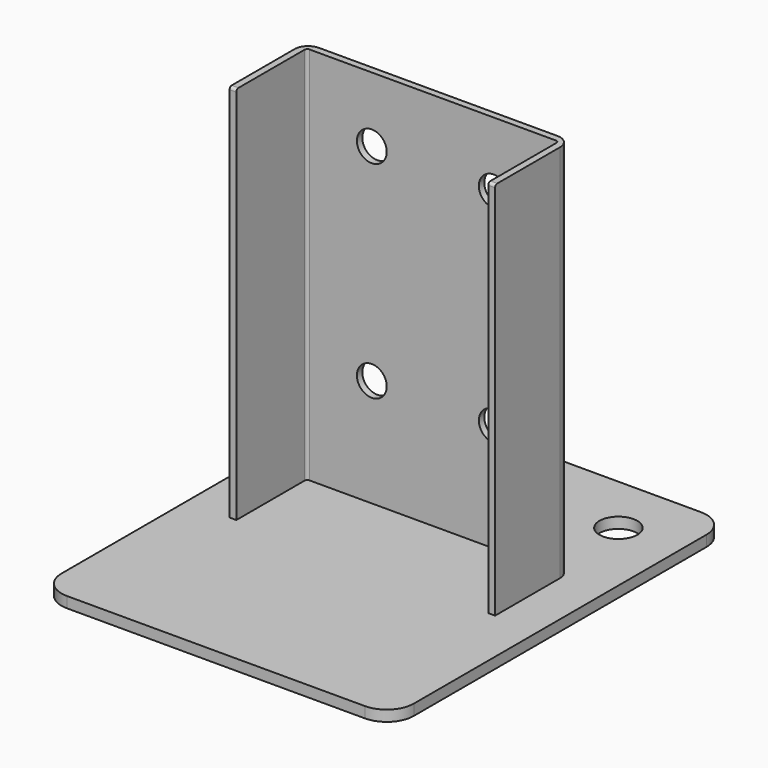
from build123d import *

# Parameters (mm, degrees)
F0_W     = 130
F0_H     = 155
F1_DEPTH = 4
F2_R     = 10
F4_DEPTH = 140
F5_R     = 5
F6_R     = 1
F7_R     = 1
F9_D     = 14
F11_D    = 11


# Not quite as in the source:
# - a feature names something its author has since deleted; it is built from what else it names


with BuildPart() as f1:
    # F0 (on Top) → F1 (new body)
    with BuildSketch(Plane.XY):
        with Locations((-65, 36.8233056366)):
            Rectangle(F0_W, F0_H)
    extrude(amount=F1_DEPTH)

    # F2
    f2_edges = [f1.edges().sort_by_distance(p)[0] for p in [
        (0, -40.676694, 2),
        (0, 114.323306, 2),
        (-130, 114.323306, 2),
        (-130, -40.676694, 2),
    ]]
    fillet(f2_edges, radius=F2_R)

    # F3 (on face) → F4 (join)
    with BuildSketch(Plane.XY.offset(4)):
        Polygon((-16, 26.8233056366), (-16, 61.8233056366), (-114, 61.8233056366), (-114, 26.8233056366), (-111.5, 26.8233056366), (-111.5, 59.3233056366), (-18.5, 59.3233056366), (-18.5, 26.8233056366), align=None)
    extrude(amount=F4_DEPTH)

    # F5
    f5_edges = [f1.edges().sort_by_distance(p)[0] for p in [
        (-114, 61.823306, 74),
        (-16, 61.823306, 74),
    ]]
    fillet(f5_edges, radius=F5_R)

    # F6
    f6_edges = [f1.edges().sort_by_distance(p)[0] for p in [
        (-18.5, 59.323306, 74),
        (-111.5, 59.323306, 74),
    ]]
    fillet(f6_edges, radius=F6_R)

    # F7
    f7_edges = [f1.edges().sort_by_distance(p)[0] for p in [
        (-112.75, 26.823306, 144),
        (-17.25, 26.823306, 144),
    ]]
    fillet(f7_edges, radius=F7_R)

    # F9 (through all)
    with Locations(Plane.XY.offset(4)):
        with Locations((-22.5, 91.8233056366), (-65, 91.8233056366), (-107.5, 91.8233056366)):
            Hole(F9_D / 2)

    # F11 (through all)
    with Locations(Plane(origin=(0, 61.8233056366, 0), x_dir=(-1, 0, 0), z_dir=(0, 1, 0))):
        with Locations((42.5, 43.8), (87.5, 43.8), (42.5, 120), (87.5, 120)):
            Hole(F11_D / 2)


solid = f1.part
